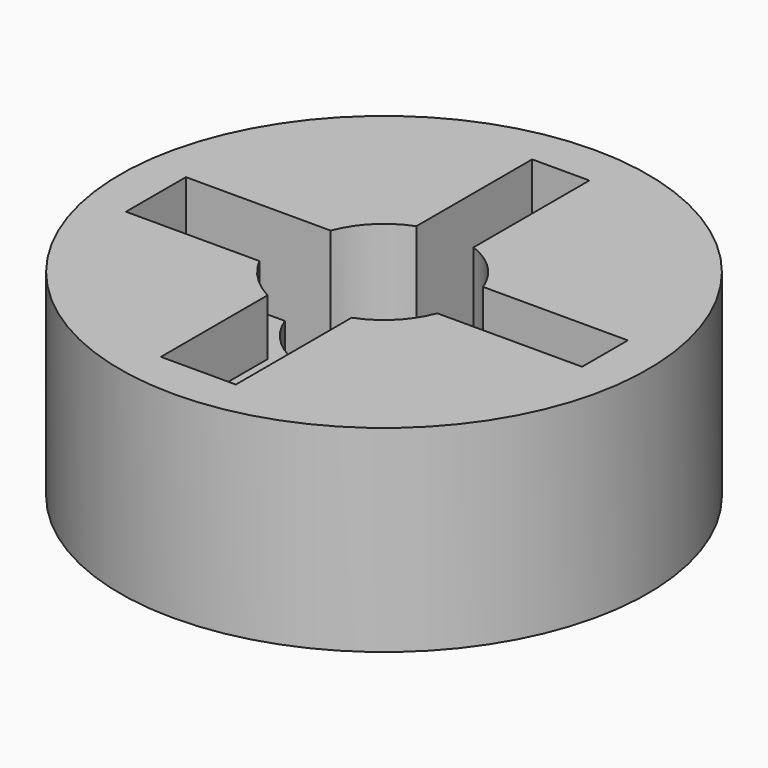
from build123d import *

# Parameters (mm, degrees)
F3_DEPTH = 13.4
F5_R     = 2.89999
F6_R     = 0.5
F7_DEPTH = 5.7


# Not quite as in the source:
# - a fillet or chamfer is up to 0.001 mm smaller than in the source, because OpenCascade refuses the exact size


with BuildPart() as f1:
    # F0 (on Right) → F1 (revolve)
    with BuildSketch(Plane.YZ):
        Polygon((1.5, 10.2), (1.5, 0), (26.75, 0), (26.75, 20), (4.125, 20), (4.125, 10.2), align=None)
    revolve(axis=Axis((0, 0, 0.3519081866), (0, 0, -1)))

    # F2 (on face) → F3 (cut)
    with BuildSketch(Plane.XY.offset(20)):
        with BuildLine():
            Line((-22.4, 2.9), (-22.4, -2.9))
            Line((-22.4, -2.9), (-7.7235030912, -2.9))
            ThreePointArc((-7.7235030912, -2.9), (-8.25, 0), (-7.7235030912, 2.9))
            Line((-7.7235030912, 2.9), (-22.4, 2.9))
        make_face()
        with BuildLine():
            ThreePointArc((-7.7235030912, 2.9), (-8.25, 0), (-7.7235030912, -2.9))
            Line((-7.7235030912, -2.9), (-2.9, -2.9))
            Line((-2.9, -2.9), (-2.9, 2.9))
            Line((-2.9, 2.9), (-7.7235030912, 2.9))
        make_face()
        with BuildLine():
            Line((-2.9, -2.9), (-7.7235030912, -2.9))
            ThreePointArc((-7.7235030912, -2.9), (-5.8336309448, -5.8336309448), (-2.9, -7.7235030912))
            Line((-2.9, -7.7235030912), (-2.9, -2.9))
        make_face()
        with BuildLine():
            Line((2.9, -2.9), (-2.9, -2.9))
            Line((-2.9, -2.9), (-2.9, -7.7235030912))
            ThreePointArc((-2.9, -7.7235030912), (0, -8.25), (2.9, -7.7235030912))
            Line((2.9, -7.7235030912), (2.9, -2.9))
        make_face()
        with BuildLine():
            ThreePointArc((-2.9, 7.7235030912), (-5.8336309448, 5.8336309448), (-7.7235030912, 2.9))
            Line((-7.7235030912, 2.9), (-2.9, 2.9))
            Line((-2.9, 2.9), (-2.9, 7.7235030912))
        make_face()
        with BuildLine():
            ThreePointArc((2.9, -7.7235030912), (0, -8.25), (-2.9, -7.7235030912))
            Line((-2.9, -7.7235030912), (-2.9, -22.4))
            Line((-2.9, -22.4), (2.9, -22.4))
            Line((2.9, -22.4), (2.9, -7.7235030912))
        make_face()
        with BuildLine():
            Line((2.9, 2.9), (2.9, -2.9))
            Line((2.9, -2.9), (7.7235030912, -2.9))
            ThreePointArc((7.7235030912, -2.9), (8.1173086828, -1.4737027342), (8.25, 0))
            ThreePointArc((8.25, 0), (8.1173086828, 1.4737027342), (7.7235030912, 2.9))
            Line((7.7235030912, 2.9), (2.9, 2.9))
        make_face()
        with BuildLine():
            Line((7.7235030912, -2.9), (2.9, -2.9))
            Line((2.9, -2.9), (2.9, -7.7235030912))
            ThreePointArc((2.9, -7.7235030912), (5.8336309448, -5.8336309448), (7.7235030912, -2.9))
        make_face()
        with BuildLine():
            Line((-2.9, 7.7235030912), (-2.9, 2.9))
            Line((-2.9, 2.9), (2.9, 2.9))
            Line((2.9, 2.9), (2.9, 7.7235030912))
            ThreePointArc((2.9, 7.7235030912), (0, 8.25), (-2.9, 7.7235030912))
        make_face()
        with BuildLine():
            Line((-2.9, 22.4), (-2.9, 7.7235030912))
            ThreePointArc((-2.9, 7.7235030912), (0, 8.25), (2.9, 7.7235030912))
            Line((2.9, 7.7235030912), (2.9, 22.4))
            Line((2.9, 22.4), (-2.9, 22.4))
        make_face()
        with BuildLine():
            ThreePointArc((8.25, 0), (8.1173086828, -1.4737027342), (7.7235030912, -2.9))
            Line((7.7235030912, -2.9), (22.4, -2.9))
            Line((22.4, -2.9), (22.4, 2.9))
            Line((22.4, 2.9), (7.7235030912, 2.9))
            ThreePointArc((7.7235030912, 2.9), (8.1173086828, 1.4737027342), (8.25, 0))
        make_face()
        with BuildLine():
            Line((2.9, 7.7235030912), (2.9, 2.9))
            Line((2.9, 2.9), (7.7235030912, 2.9))
            ThreePointArc((7.7235030912, 2.9), (5.8336309448, 5.8336309448), (2.9, 7.7235030912))
        make_face()
    extrude(amount=-F3_DEPTH, mode=Mode.SUBTRACT)

    # F5 (radius 2.9 in the source; OpenCascade refuses exactly that, so slightly less here)
    f5_edges = [f1.edges().sort_by_distance(p)[0] for p in [
        (2.9, 2.9, 8.4),
        (-2.9, -2.9, 8.4),
        (-2.9, 2.9, 8.4),
        (2.9, -2.9, 8.4),
    ]]
    fillet(f5_edges, radius=F5_R)

    # F6
    f6_edges = [f1.edges().sort_by_distance(p)[0] for p in [
        (-2.050613, -2.050613, 6.6),
        (-2.050613, -2.050613, 10.2),
    ]]
    fillet(f6_edges, radius=F6_R)

    # F4 (on face) → F7 (cut)
    with BuildSketch(Plane.XY.offset(20)):
        with BuildLine():
            Line((-4.7, -8.883270794), (-4.7, -22.4))
            Line((-4.7, -22.4), (-2.9, -22.4))
            Line((-2.9, -22.4), (-2.9, -7.7235030912))
            ThreePointArc((-2.9, -7.7235030912), (-5.8336309448, -5.8336309448), (-7.7235030912, -2.9))
            Line((-7.7235030912, -2.9), (-22.4, -2.9))
            Line((-22.4, -2.9), (-22.4, -4.7))
            Line((-22.4, -4.7), (-8.883270794, -4.7))
            ThreePointArc((-8.883270794, -4.7), (-7.1064231509, -7.1064231509), (-4.7, -8.883270794))
        make_face()
    extrude(amount=-F7_DEPTH, mode=Mode.SUBTRACT)


solid = f1.part
